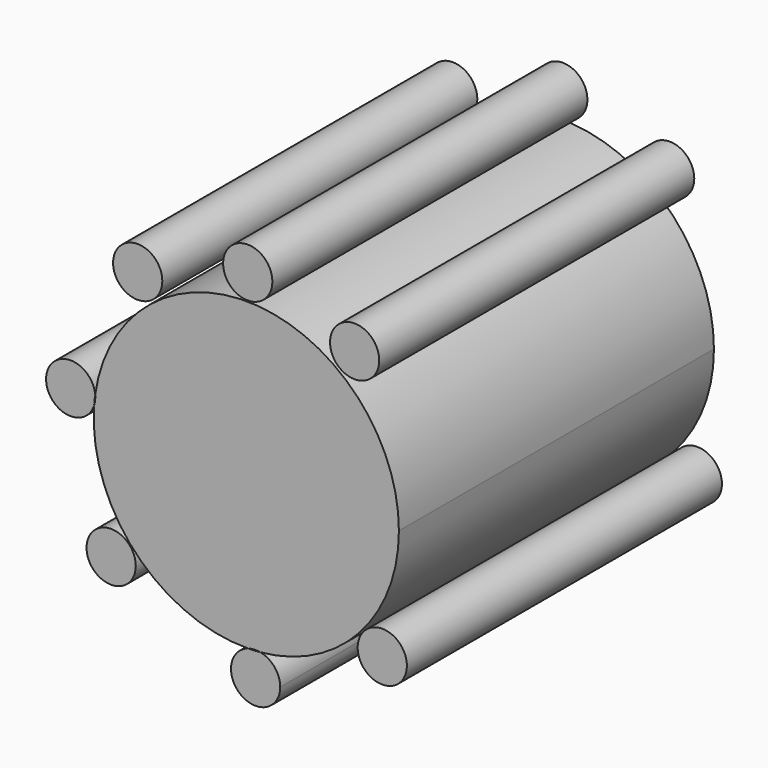
from build123d import *

# Parameters (mm, degrees)
F1_DEPTH = 80
F0_R     = 5


with BuildPart() as f1:
    # F0 (on Front) → F1 (new body)
    with BuildSketch(Plane.XZ):
        with BuildLine():
            ThreePointArc((1.2717998454, -30.8674716863), (21.3187032133, -20.8834130919), (29.4083767724, 0))
            ThreePointArc((29.4083767724, 0), (0.5616103001, 30.9251287043), (-32.2924997034, 4.2960660629))
            ThreePointArc((-32.2924997034, 4.2960660629), (-32.274802335, 4.05373467), (-32.2688985649, 3.810829655))
            ThreePointArc((-32.2688985649, 3.810829655), (-32.3288490863, 3.0388768397), (-32.5072630246, 2.2854356139))
            ThreePointArc((-32.5072630246, 2.2854356139), (-24.1679170215, -21.2440805528), (-1.1884477149, -30.997378107))
            ThreePointArc((-1.1884477149, -30.997378107), (0.0335496433, -30.7785217279), (1.2717998454, -30.8674716863))
        make_face()
    extrude(amount=F1_DEPTH)


with BuildPart() as f1b:
    # F0 (on Front) → F1, piece 2 (new body)
    with BuildSketch(Plane.XZ):
        with BuildLine():
            ThreePointArc((-32.5072630246, 2.2854356139), (-32.4162793992, 3.2925023768), (-32.2924997034, 4.2960660629))
            ThreePointArc((-32.2924997034, 4.2960660629), (-42.2406173023, 4.3418784255), (-32.5072630246, 2.2854356139))
        make_face()
    extrude(amount=F1_DEPTH)


with BuildPart() as f1c:
    # F0 (on Front) → F1, piece 3 (new body)
    with BuildSketch(Plane.XZ):
        with BuildLine():
            ThreePointArc((5.2971932426, -35.771566095), (4.1619722152, -32.5992666935), (1.2717998454, -30.8674716863))
            ThreePointArc((1.2717998454, -30.8674716863), (0.0429670879, -30.9568750765), (-1.1884477149, -30.997378107))
            ThreePointArc((-1.1884477149, -30.997378107), (-2.6669082413, -39.7982399574), (5.2971932426, -35.771566095))
        make_face()
    extrude(amount=F1_DEPTH)


with BuildPart() as f1d:
    # F0 (on Front) → F1, piece 4 (new body)
    with BuildSketch(Plane.XZ):
        with Locations((-23.6584274116, 29.0477543936)):
            Circle(F0_R)
    extrude(amount=F1_DEPTH)


with BuildPart() as f1e:
    # F0 (on Front) → F1, piece 5 (new body)
    with BuildSketch(Plane.XZ):
        with Locations((-29.0477543936, -23.6584274116)):
            Circle(F0_R)
    extrude(amount=F1_DEPTH)


with BuildPart() as f1f:
    # F0 (on Front) → F1, piece 6 (new body)
    with BuildSketch(Plane.XZ):
        with Locations((20.4142962822, 29.1755563039)):
            Circle(F0_R)
    extrude(amount=F1_DEPTH)


with BuildPart() as f1g:
    # F0 (on Front) → F1, piece 7 (new body)
    with BuildSketch(Plane.XZ):
        with Locations((26.028754213, -23.5964425308)):
            Circle(F0_R)
    extrude(amount=F1_DEPTH)


with BuildPart() as f1h:
    # F0 (on Front) → F1, piece 8 (new body)
    with BuildSketch(Plane.XZ):
        with Locations((-1.2987746409, 36.2154911415)):
            Circle(F0_R)
    extrude(amount=F1_DEPTH)


solid = Compound([f1.part, f1b.part, f1c.part, f1d.part, f1e.part, f1f.part, f1g.part, f1h.part])
